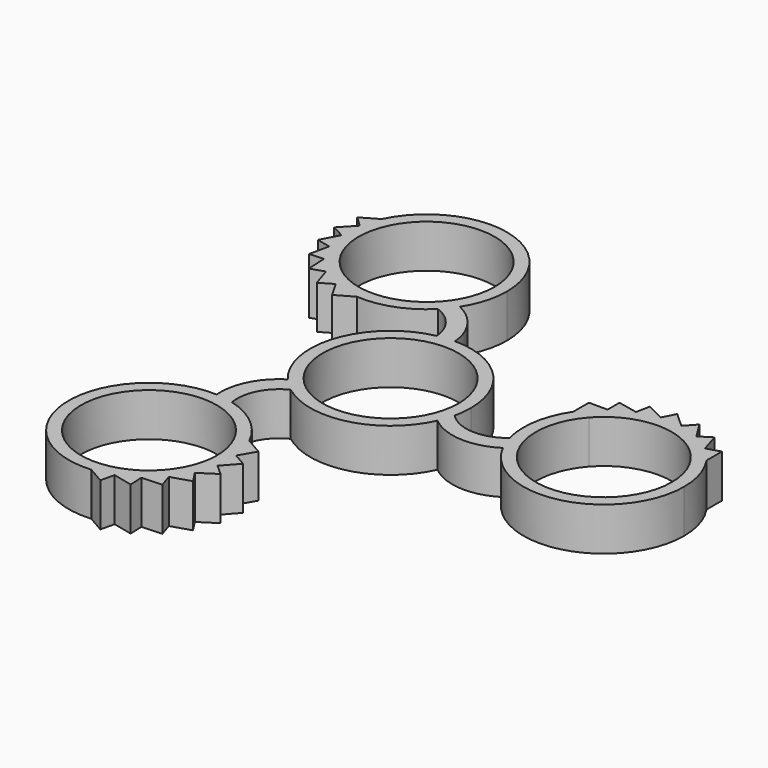
from build123d import *

# Parameters (mm, degrees)
F0_R     = 11
F1_DEPTH = 7


# Not quite as in the source:
# - a feature names something its author has since deleted; it is built from what else it names


with BuildPart() as f1:
    # F0 (on Top) → F1 (new body)
    with BuildSketch(Plane.XY):
        with BuildLine():
            ThreePointArc((42.7437567563, 7.2828891618), (44.7878891013, 3.8934994337), (45.5, 0))
            ThreePointArc((45.5, 0), (30.6065005663, -10.2878891013), (26.2562432437, 7.2828891618))
            Line((26.2562432437, 7.2828891618), (23.7315495331, 7.2828891618))
            ThreePointArc((23.7315495331, 7.2828891618), (21.6811026337, 2.16237608), (21.9383596578, -3.3474157066))
            ThreePointArc((21.9383596578, -3.3474157066), (22.3825285727, -4.708172279), (22.9736088848, -6.0118472917))
            ThreePointArc((22.9736088848, -6.0118472917), (37.5949083591, -12.6262243861), (47.5, 0))
            ThreePointArc((47.5, 0), (46.9295988686, 3.8085524764), (45.2684504669, 7.2828891618))
            Line((45.2684504669, 7.2828891618), (42.7437567563, 7.2828891618))
        make_face()
        with BuildLine():
            ThreePointArc((26.2562432437, 7.2828891618), (34.5, 11), (42.7437567563, 7.2828891618))
            Line((42.7437567563, 7.2828891618), (45.2684504669, 7.2828891618))
            ThreePointArc((45.2684504669, 7.2828891618), (45.2378577502, 7.3279199597), (45.207076728, 7.3728222508))
            ThreePointArc((45.207076728, 7.3728222508), (44.1835161526, 8.6734949658), (43.0029894611, 9.8335736243))
            ThreePointArc((43.0029894611, 9.8335736243), (41.6158857772, 10.879529843), (40.1017032771, 11.7311943295))
            ThreePointArc((40.1017032771, 11.7311943295), (38.4874829399, 12.3733576609), (36.8020522674, 12.7945517842))
            ThreePointArc((36.8020522674, 12.7945517842), (35.0755104688, 12.9872548177), (33.3386909351, 12.9480253806))
            ThreePointArc((33.3386909351, 12.9480253806), (31.6226106019, 12.6775640504), (29.9579160343, 12.1807008521))
            ThreePointArc((29.9579160343, 12.1807008521), (28.2960857777, 11.4241607272), (26.7566463688, 10.442244708))
            ThreePointArc((26.7566463688, 10.442244708), (25.1102659991, 8.9907116177), (23.7315495331, 7.2828891618))
            Line((23.7315495331, 7.2828891618), (26.2562432437, 7.2828891618))
        make_face()
        with BuildLine():
            Line((23.7315495331, 10.442244708), (23.7315495331, 7.2828891618))
            ThreePointArc((23.7315495331, 7.2828891618), (25.1102659991, 8.9907116177), (26.7566463688, 10.442244708))
            Line((26.7566463688, 10.442244708), (23.7315495331, 10.442244708))
        make_face()
        with BuildLine():
            ThreePointArc((43.0029894611, 9.8335736243), (44.1835161526, 8.6734949658), (45.207076728, 7.3728222508))
            Line((45.207076728, 7.3728222508), (45.207076728, 10.5051657741))
            Line((45.207076728, 10.5051657741), (43.0029894611, 9.8335736243))
        make_face()
        with BuildLine():
            Line((26.7566463688, 12.8468079515), (26.7566463688, 10.442244708))
            ThreePointArc((26.7566463688, 10.442244708), (28.2960857777, 11.4241607272), (29.9579160343, 12.1807008521))
            Line((29.9579160343, 12.1807008521), (26.7566463688, 12.8468079515))
        make_face()
        with BuildLine():
            ThreePointArc((22.9736088848, -6.0118472917), (22.3825285727, -4.708172279), (21.9383596578, -3.3474157066))
            ThreePointArc((21.9383596578, -3.3474157066), (17.3922362251, -4.9568983328), (12.9232065297, -3.1443183566))
            ThreePointArc((12.9232065297, -3.1443183566), (12.7963014273, -3.0234598131), (12.6725554503, -2.8993686138))
            ThreePointArc((12.6725554503, -2.8993686138), (12.3249994875, -4.1345359635), (11.8573707885, -5.3294237947))
            ThreePointArc((11.8573707885, -5.3294237947), (17.3029186127, -7.5043480898), (22.9736088848, -6.0118472917))
        make_face()
        with BuildLine():
            ThreePointArc((40.1017032771, 11.7311943295), (41.6158857772, 10.879529843), (43.0029894611, 9.8335736243))
            Line((43.0029894611, 9.8335736243), (42.0499218924, 12.9614304542))
            Line((42.0499218924, 12.9614304542), (40.1017032771, 11.7311943295))
        make_face()
        with BuildLine():
            Line((30.4272975488, 14.4365194817), (29.9579160343, 12.1807008521))
            ThreePointArc((29.9579160343, 12.1807008521), (31.6226106019, 12.6775640504), (33.3386909351, 12.9480253806))
            Line((33.3386909351, 12.9480253806), (30.4272975488, 14.4365194817))
        make_face()
        with BuildLine():
            ThreePointArc((-7.9002965036, -10.3240164255), (3.1860787986, -12.603527359), (11.8573707885, -5.3294237947))
            ThreePointArc((11.8573707885, -5.3294237947), (12.3249994875, -4.1345359635), (12.6725554503, -2.8993686138))
            ThreePointArc((12.6725554503, -2.8993686138), (12.9178794865, -1.4589001244), (13, 0))
            ThreePointArc((13, 0), (9.2025905119, 9.1821744631), (0.0288726353, 12.9999679373))
            ThreePointArc((0.0288726353, 12.9999679373), (-1.3452884897, 12.9302049048), (-2.7043793136, 12.715594069))
            ThreePointArc((-2.7043793136, 12.715594069), (-12.2885029344, 4.2417797718), (-9.9723418366, -8.339808049))
            ThreePointArc((-9.9723418366, -8.339808049), (-8.9912218875, -9.3892453887), (-7.9002965036, -10.3240164255))
        make_face()
        Circle(F0_R, mode=Mode.SUBTRACT)
        with BuildLine():
            ThreePointArc((36.8020522674, 12.7945517842), (38.4874829399, 12.3733576609), (40.1017032771, 11.7311943295))
            Line((40.1017032771, 11.7311943295), (38.3558547697, 14.4959437083))
            Line((38.3558547697, 14.4959437083), (36.8020522674, 12.7945517842))
        make_face()
        with BuildLine():
            Line((34.3875787435, 14.9995787095), (33.3386909351, 12.9480253806))
            ThreePointArc((33.3386909351, 12.9480253806), (35.0755104688, 12.9872548177), (36.8020522674, 12.7945517842))
            Line((36.8020522674, 12.7945517842), (34.3875787435, 14.9995787095))
        make_face()
        with BuildLine():
            ThreePointArc((-11.5709617185, -17.6259791714), (-10.9561833098, -13.361430461), (-7.9002965036, -10.3240164255))
            ThreePointArc((-7.9002965036, -10.3240164255), (-8.9912218875, -9.3892453887), (-9.9723418366, -8.339808049))
            ThreePointArc((-9.9723418366, -8.339808049), (-13.420933272, -12.1469092689), (-14.3960517714, -17.1903155086))
            ThreePointArc((-14.3960517714, -17.1903155086), (-12.971495936, -17.3302624491), (-11.5709617185, -17.6259791714))
        make_face()
        with BuildLine():
            ThreePointArc((-3.2614425902, -24.4940795914), (-6.6707135497, -20.1580839465), (-11.5709617185, -17.6259791714))
            ThreePointArc((-11.5709617185, -17.6259791714), (-12.971495936, -17.3302624491), (-14.3960517714, -17.1903155086))
            ThreePointArc((-14.3960517714, -17.1903155086), (-27.9515414405, -30.3617633129), (-14.0298930571, -43.1455829188))
            Line((-14.0298930571, -43.1455829188), (-12.7675462018, -40.9591340287))
            ThreePointArc((-12.7675462018, -40.9591340287), (-24.4791142923, -24.6783866742), (-4.5237894455, -26.6805284815))
            Line((-4.5237894455, -26.6805284815), (-3.2614425902, -24.4940795914))
        make_face()
        with BuildLine():
            ThreePointArc((-2.7043793136, 12.715594069), (-1.3452884897, 12.9302049048), (0.0288726353, 12.9999679373))
            ThreePointArc((0.0288726353, 12.9999679373), (-1.6510654504, 17.6006925658), (-5.3920588945, 20.7619940589))
            ThreePointArc((-5.3920588945, 20.7619940589), (-6.2255344178, 19.5982659865), (-7.1818997204, 18.5332261365))
            ThreePointArc((-7.1818997204, 18.5332261365), (-4.0898299015, 16.2811568981), (-2.7043793136, 12.715594069))
        make_face()
        with BuildLine():
            Line((-0.5253604276, -26.0737573645), (-3.2614425902, -24.4940795914))
            ThreePointArc((-3.2614425902, -24.4940795914), (-2.4717831912, -26.5419943035), (-2.0379088454, -28.6935680732))
            Line((-2.0379088454, -28.6935680732), (-0.5253604276, -26.0737573645))
        make_face()
        with BuildLine():
            ThreePointArc((-2.0379088454, -28.6935680732), (-2.4717831912, -26.5419943035), (-3.2614425902, -24.4940795914))
            Line((-3.2614425902, -24.4940795914), (-4.5237894455, -26.6805284815))
            ThreePointArc((-4.5237894455, -26.6805284815), (-4.0965118208, -28.4063115428), (-3.9528348507, -30.1783866742))
            ThreePointArc((-3.9528348507, -30.1783866742), (-6.4370208809, -37.1412102704), (-12.7675462018, -40.9591340287))
            Line((-12.7675462018, -40.9591340287), (-14.0298930571, -43.1455829188))
            ThreePointArc((-14.0298930571, -43.1455829188), (-13.9755988838, -43.141604248), (-13.9213218479, -43.1373982463))
            ThreePointArc((-13.9213218479, -43.1373982463), (-12.283125947, -42.9013051432), (-10.6882050126, -42.4589783678))
            ThreePointArc((-10.6882050126, -42.4589783678), (-9.088828514, -41.7806894492), (-7.5941741832, -40.8952011814))
            ThreePointArc((-7.5941741832, -40.8952011814), (-6.2309342562, -39.8183270277), (-5.0234541092, -38.5692983107))
            ThreePointArc((-5.0234541092, -38.5692983107), (-3.9932974875, -37.1704207692), (-3.1588614098, -35.6466762127))
            ThreePointArc((-3.1588614098, -35.6466762127), (-2.5350476259, -34.0252763841), (-2.132996494, -32.3351769998))
            ThreePointArc((-2.132996494, -32.3351769998), (-1.9979535576, -31.2605376256), (-1.9528348507, -30.1783866742))
            ThreePointArc((-1.9528348507, -30.1783866742), (-1.9741207759, -29.4347597747), (-2.0379088454, -28.6935680732))
        make_face()
        with BuildLine():
            ThreePointArc((-7.1818997204, 18.5332261365), (-6.2255344178, 19.5982659865), (-5.3920588945, 20.7619940589))
            ThreePointArc((-5.3920588945, 20.7619940589), (-3.8795816786, 24.105375001), (-3.3616669305, 27.7382179327))
            ThreePointArc((-3.3616669305, 27.7382179327), (-13.4451706923, 40.40684255), (-28.0530591909, 33.4225250156))
            Line((-28.0530591909, 33.4225250156), (-26.7907123357, 31.2360761255))
            ThreePointArc((-26.7907123357, 31.2360761255), (-14.589591799, 38.5945409626), (-5.3616669305, 27.7382179327))
            ThreePointArc((-5.3616669305, 27.7382179327), (-9.3988433343, 19.2224039629), (-18.5469555793, 16.9574705783))
            Line((-18.5469555793, 16.9574705783), (-17.2846087241, 14.7710216882))
            ThreePointArc((-17.2846087241, 14.7710216882), (-11.8248908651, 15.555539125), (-7.1818997204, 18.5332261365))
        make_face()
        with BuildLine():
            Line((0.0445040084, -29.8958496949), (-2.0379088454, -28.6935680732))
            ThreePointArc((-2.0379088454, -28.6935680732), (-1.9741207759, -29.4347597747), (-1.9528348507, -30.1783866742))
            ThreePointArc((-1.9528348507, -30.1783866742), (-1.9979535576, -31.2605376256), (-2.132996494, -32.3351769998))
            Line((-2.132996494, -32.3351769998), (0.0445040084, -29.8958496949))
        make_face()
        with BuildLine():
            Line((-20.0206908867, 13.191343915), (-17.2846087241, 14.7710216882))
            ThreePointArc((-17.2846087241, 14.7710216882), (-19.452984589, 15.1111139443), (-21.5332393046, 15.8111546236))
            Line((-21.5332393046, 15.8111546236), (-20.0206908867, 13.191343915))
        make_face()
        with BuildLine():
            ThreePointArc((-21.5332393046, 15.8111546236), (-19.452984589, 15.1111139443), (-17.2846087241, 14.7710216882))
            Line((-17.2846087241, 14.7710216882), (-18.5469555793, 16.9574705783))
            ThreePointArc((-18.5469555793, 16.9574705783), (-25.8879463721, 22.2382179327), (-26.7907123357, 31.2360761255))
            Line((-26.7907123357, 31.2360761255), (-28.0530591909, 33.4225250156))
            ThreePointArc((-28.0530591909, 33.4225250156), (-28.0767606476, 33.3735155468), (-28.1002566612, 33.3244072541))
            ThreePointArc((-28.1002566612, 33.3244072541), (-28.7148919868, 31.7876414359), (-29.1292862296, 30.185236002))
            ThreePointArc((-29.1292862296, 30.185236002), (-29.3415590444, 28.4609908647), (-29.322030875, 26.7238381104))
            ThreePointArc((-29.322030875, 26.7238381104), (-29.0710504648, 25.0048006254), (-28.5930999393, 23.334577785))
            ThreePointArc((-28.5930999393, 23.334577785), (-27.8967147624, 21.74299721), (-26.9943313064, 20.2584820906))
            ThreePointArc((-26.9943313064, 20.2584820906), (-25.9020647571, 18.9075435922), (-24.6394213214, 17.7143074062))
            ThreePointArc((-24.6394213214, 17.7143074062), (-23.153323226, 16.6533902497), (-21.5332393046, 15.8111546236))
        make_face()
        with BuildLine():
            ThreePointArc((-10.6882050126, -42.4589783678), (-12.283125947, -42.9013051432), (-13.9213218479, -43.1373982463))
            Line((-13.9213218479, -43.1373982463), (-11.2086327833, -44.703570008))
            Line((-11.2086327833, -44.703570008), (-10.6882050126, -42.4589783678))
        make_face()
        with BuildLine():
            Line((-23.6156521584, 14.6088730019), (-21.5332393046, 15.8111546236))
            ThreePointArc((-21.5332393046, 15.8111546236), (-23.153323226, 16.6533902497), (-24.6394213214, 17.7143074062))
            Line((-24.6394213214, 17.7143074062), (-23.6156521584, 14.6088730019))
        make_face()
        with BuildLine():
            ThreePointArc((-7.5941741832, -40.8952011814), (-9.088828514, -41.7806894492), (-10.6882050126, -42.4589783678))
            Line((-10.6882050126, -42.4589783678), (-7.5028677542, -43.1975260567))
            Line((-7.5028677542, -43.1975260567), (-7.5941741832, -40.8952011814))
        make_face()
        with BuildLine():
            Line((-0.4140910118, -33.8695826303), (-2.132996494, -32.3351769998))
            ThreePointArc((-2.132996494, -32.3351769998), (-2.5350476259, -34.0252763841), (-3.1588614098, -35.6466762127))
            Line((-3.1588614098, -35.6466762127), (-0.4140910118, -33.8695826303))
        make_face()
        with BuildLine():
            ThreePointArc((-29.1292862296, 30.185236002), (-28.7148919868, 31.7876414359), (-28.1002566612, 33.3244072541))
            Line((-28.1002566612, 33.3244072541), (-30.8129457258, 31.7582354924))
            Line((-30.8129457258, 31.7582354924), (-29.1292862296, 30.185236002))
        make_face()
        with BuildLine():
            Line((-26.8277083182, 16.9928944072), (-24.6394213214, 17.7143074062))
            ThreePointArc((-24.6394213214, 17.7143074062), (-25.9020647571, 18.9075435922), (-26.9943313064, 20.2584820906))
            Line((-26.9943313064, 20.2584820906), (-26.8277083182, 16.9928944072))
        make_face()
        with BuildLine():
            ThreePointArc((-5.0234541092, -38.5692983107), (-6.2309342562, -39.8183270277), (-7.5941741832, -40.8952011814))
            Line((-7.5941741832, -40.8952011814), (-4.3269067323, -40.7656267122))
            Line((-4.3269067323, -40.7656267122), (-5.0234541092, -38.5692983107))
        make_face()
        with BuildLine():
            Line((-1.906608014, -37.5808163649), (-3.1588614098, -35.6466762127))
            ThreePointArc((-3.1588614098, -35.6466762127), (-3.9932974875, -37.1704207692), (-5.0234541092, -38.5692983107))
            Line((-5.0234541092, -38.5692983107), (-1.906608014, -37.5808163649))
        make_face()
        with BuildLine():
            ThreePointArc((-29.322030875, 26.7238381104), (-29.3415590444, 28.4609908647), (-29.1292862296, 30.185236002))
            Line((-29.1292862296, 30.185236002), (-31.3615559194, 27.795926861))
            Line((-31.3615559194, 27.795926861), (-29.322030875, 26.7238381104))
        make_face()
        with BuildLine():
            Line((-29.2954725106, 20.1410689139), (-26.9943313064, 20.2584820906))
            ThreePointArc((-26.9943313064, 20.2584820906), (-27.8967147624, 21.74299721), (-28.5930999393, 23.334577785))
            Line((-28.5930999393, 23.334577785), (-29.2954725106, 20.1410689139))
        make_face()
        with BuildLine():
            ThreePointArc((-28.5930999393, 23.334577785), (-29.0710504648, 25.0048006254), (-29.322030875, 26.7238381104))
            Line((-29.322030875, 26.7238381104), (-30.8434498185, 23.8295142624))
            Line((-30.8434498185, 23.8295142624), (-28.5930999393, 23.334577785))
        make_face()
    extrude(amount=F1_DEPTH)


solid = f1.part
